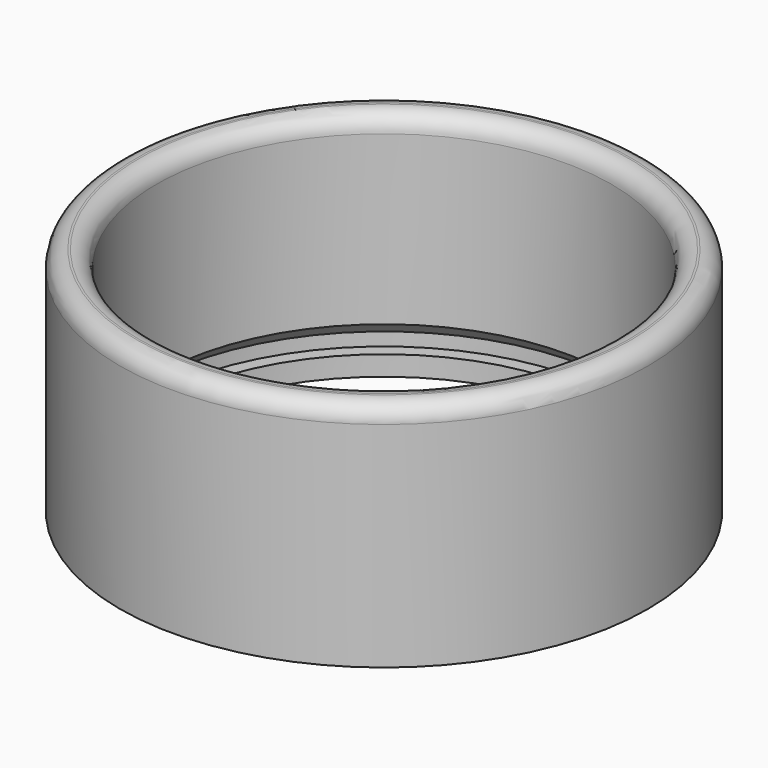
from build123d import *

# Parameters (mm, degrees)
F0_R     = 20
F0_R_2   = 17.25
F1_DEPTH = 1.5
F2_R     = 20
F2_R_2   = 18.25
F3_DEPTH = 1
F4_R     = 20
F4_R_2   = 17.25
F5_DEPTH = 15
F6_R     = 1.3
F7_SIZE  = 0.99999


# Not quite as in the source:
# - a fillet or chamfer is up to 0.001 mm smaller than in the source, because OpenCascade refuses the exact size


with BuildPart() as f1:
    # F0 (on Top) → F1 (new body)
    with BuildSketch(Plane.XY):
        Circle(F0_R)
        Circle(F0_R_2, mode=Mode.SUBTRACT)
    extrude(amount=F1_DEPTH)

    # F2 (on face) → F3 (join)
    with BuildSketch(Plane.XY.offset(1.5)):
        Circle(F2_R)
        Circle(F2_R_2, mode=Mode.SUBTRACT)
    extrude(amount=F3_DEPTH)

    # F4 (on face) → F5 (join)
    with BuildSketch(Plane.XY.offset(2.5)):
        Circle(F4_R)
        Circle(F4_R_2, mode=Mode.SUBTRACT)
    extrude(amount=F5_DEPTH)

    # F6
    f6_edges = [f1.edges().sort_by_distance(p)[0] for p in [
        (-17.25, 0, 17.5),
        (-20, 0, 17.5),
    ]]
    fillet(f6_edges, radius=F6_R)

    # F7 (size 1 in the source; OpenCascade refuses exactly that, so slightly less here)
    f7_edges = [f1.edges().sort_by_distance(p)[0] for p in [
        (-17.25, 0, 2.5),
    ]]
    chamfer(f7_edges, length=F7_SIZE)


solid = f1.part
